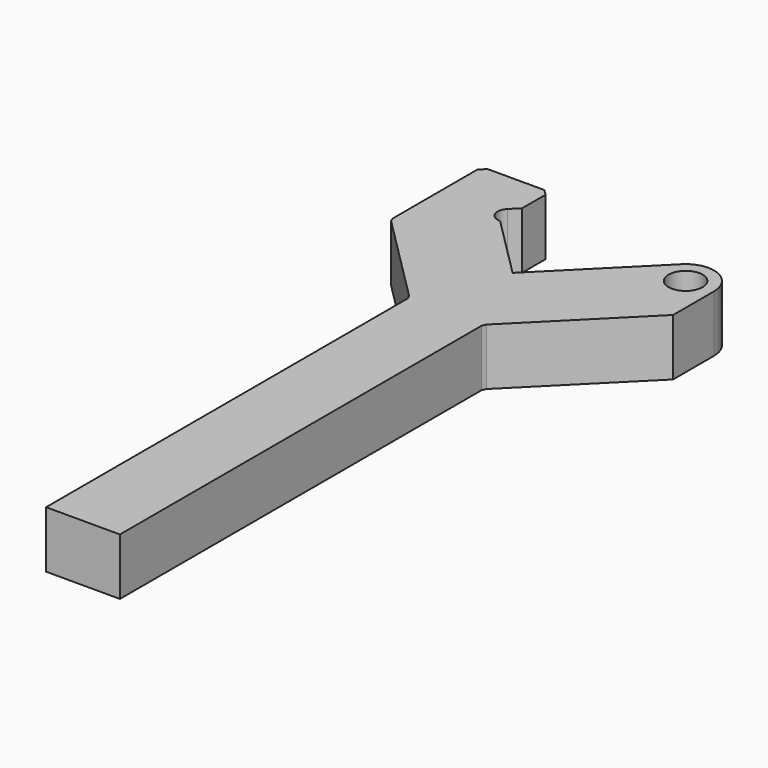
from build123d import *

# Parameters (mm, degrees)
F0_R        = 3
F1_DEPTH    = 10
F2_R        = 5
F3_R        = 4.99999
F4_T1_DEPTH = 10
F4_T3_DEPTH = 15.1433659759
F4_T5_DEPTH = 12.2571417204


# Not quite as in the source:
# - a fillet or chamfer that OpenCascade refuses, or shapes differently, is made with other operations: its cross-section is extruded or revolved along the edge and cut away or added
# - a fillet or chamfer is up to 0.001 mm smaller than in the source, because OpenCascade refuses the exact size


with BuildPart() as f1:
    # F0 (on Top) → F1 (new body)
    with BuildSketch(Plane.XY):
        with BuildLine():
            Line((18, 18), (0, 0))
            Line((0, 0), (-11, 11))
            ThreePointArc((-11, 11), (-12.8659446975, 12.2241130817), (-12.4367385267, 14.4140867148))
            Line((-12.4367385267, 14.4140867148), (-11, 15.8508252416))
            Line((-11, 15.8508252416), (-11, 21.9997463049))
            Line((-11, 21.9997463049), (-23, 21.9997463049))
            Line((-23, 21.9997463049), (-23, 1.9289321881))
            Line((-23, 1.9289321881), (-6.5, -14.5710678119))
            Line((-6.5, -14.5710678119), (-6.5, -94.5710678119))
            Line((-6.5, -94.5710678119), (6.5, -94.5710678119))
            Line((6.5, -94.5710678119), (6.5, -14.5710678119))
            Line((6.5, -14.5710678119), (25.0710678119, 4))
            Line((25.0710678119, 4), (25.0710678119, 18))
            Line((25.0710678119, 18), (18, 18))
        make_face()
        with Locations((20.0710678119, 13)):
            Circle(F0_R, mode=Mode.SUBTRACT)
    extrude(amount=F1_DEPTH)

    # F2
    f2_edges = [f1.edges().sort_by_distance(p)[0] for p in [
        (18, 18, 5),
    ]]
    fillet(f2_edges, radius=F2_R)

    # F3 (radius 5 in the source; OpenCascade refuses exactly that, so slightly less here)
    f3_edges = [f1.edges().sort_by_distance(p)[0] for p in [
        (25.071068, 18, 5),
    ]]
    fillet(f3_edges, radius=F3_R)

    # F4: chamfer of 1 on 5 edges, made by hand

    # F4_s2 → F4_t1 (join)
    with BuildSketch(Plane.XY):
        Polygon((-6.5, -14.9852813742), (-6.7928932188, -14.2781745931), (-6.5, -14.5710678119), align=None)
        Polygon((6.7928932188, -14.2781745931), (6.5, -14.9852813742), (6.5, -14.5710678119), align=None)
    extrude(amount=F4_T1_DEPTH)

    # F4_s4 → F4_t3 (cut)
    with BuildSketch(Plane.XY.offset(-2.571682988)):
        Polygon((-11, 20.9997463049), (-12, 21.9997463049), (-11, 21.9997463049), align=None)
        Polygon((-22, 21.9997463049), (-23, 20.9997463049), (-23, 21.9997463049), align=None)
    extrude(amount=F4_T3_DEPTH, mode=Mode.SUBTRACT)

    # F4_s6 → F4_t5 (cut)
    with BuildSketch(Plane.XY.offset(-1.1285708602)):
        Polygon((-22.7071067812, 1.6360389693), (-23, 2.3431457505), (-23, 1.9289321881), align=None)
    extrude(amount=F4_T5_DEPTH, mode=Mode.SUBTRACT)


solid = f1.part
